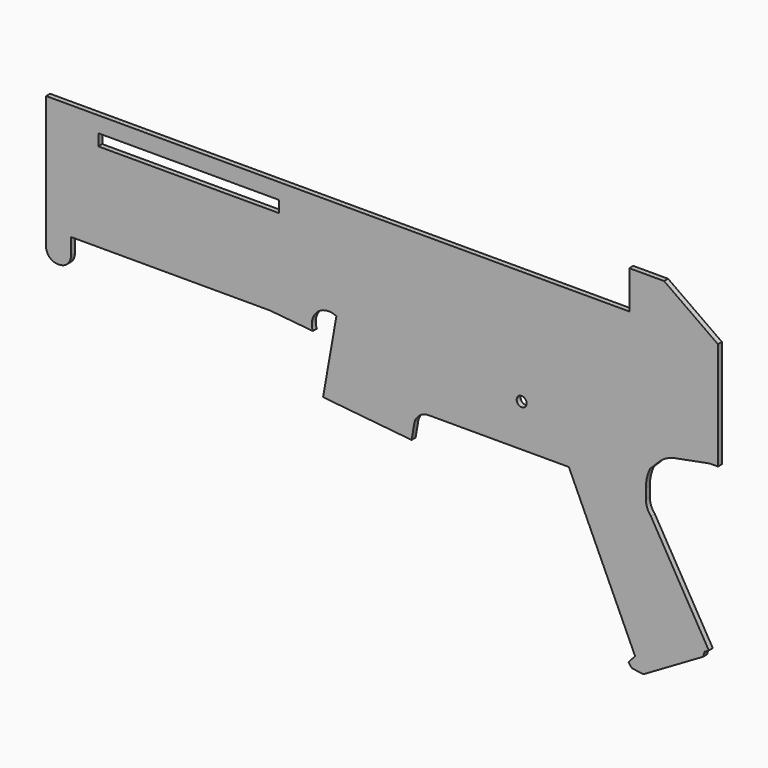
from build123d import *

# Parameters (mm, degrees)
F0_W     = 109
F0_H     = 7
F0_R     = 3
F1_DEPTH = 3


# Not quite as in the source:
# - a feature names something its author has since deleted; it is built from what else it names


with BuildPart() as f1:
    # F0 (on Front) → F1 (new body)
    with BuildSketch(Plane.XZ):
        with BuildLine():
            Line((48.4662945779, -65), (53.4662945779, -65))
            Line((53.4662945779, -65), (53.4662945779, 0))
            Line((53.4662945779, 0), (20.9662945779, 22.9999753031))
            Line((20.9662945779, 22.9999753031), (-0.0337054221, 22.9999753031))
            Line((-0.0337054221, 22.9999753031), (0, 0))
            Line((0, 0), (-352, 0))
            Line((-352, 0), (-352, -39))
            Line((-352, -39), (-352, -55.5))
            Line((-352, -55.5), (-352, -80))
            ThreePointArc((-352, -80), (-349.9497474683, -84.9497474683), (-345, -87))
            Line((-345, -87), (-344, -87))
            ThreePointArc((-344, -87), (-339.0502525317, -84.9497474683), (-337, -80))
            Line((-337, -80), (-337, -70))
            Line((-337, -70), (-217, -70))
            Line((-217, -70), (-191, -72.5))
            ThreePointArc((-191, -72.5), (-188.1802970177, -61.3925278998), (-176.8015588718, -60.0320207981))
            Line((-176.8015588718, -60.0320207981), (-179, -72.5))
            Line((-179, -72.5), (-184.8187903634, -105.5))
            Line((-184.8187903634, -105.5), (-181.3187903634, -106))
            Line((-181.3187903634, -106), (-131.43, -111.007))
            Line((-131.43, -111.007), (-129.63038537, -100.8008782668))
            ThreePointArc((-129.63038537, -100.8008782668), (-126.3267144318, -96.2419842885), (-120.9729076822, -94.5))
            Line((-120.9729076822, -94.5), (-97.5, -94.5))
            Line((-97.5, -94.5), (-36.5, -94.5))
            Line((-36.5, -94.5), (3.4662945779, -182))
            Line((3.4662945779, -182), (-0.5337054221, -186.5))
            Line((-0.5337054221, -186.5), (1.4662945779, -189))
            Line((1.4662945779, -189), (8.4662945779, -190))
            Line((8.4662945779, -190), (44.4662945779, -169))
            Line((44.4662945779, -169), (45.4662945779, -166))
            Line((45.4662945779, -166), (47.9662945779, -164.5))
            Line((47.9662945779, -164.5), (12.9662945779, -104.5))
            ThreePointArc((12.9662945779, -104.5), (10.7409562508, -100.7720018727), (9.9662945779, -96.5))
            Line((9.9662945779, -96.5), (9.9662945779, -90.5))
            ThreePointArc((9.9662945779, -90.5), (10.599163398, -84.8597429137), (12.4662945779, -79.5))
            Line((12.4662945779, -79.5), (18.4662945779, -73.5))
            ThreePointArc((18.4662945779, -73.5), (22.6544664529, -70.6263437501), (27.4662945779, -69))
            Line((27.4662945779, -69), (48.4662945779, -65))
        make_face()
        with Locations((-266, -13)):
            Rectangle(F0_W, F0_H, mode=Mode.SUBTRACT)
        with Locations((-65, -69)):
            Circle(F0_R, mode=Mode.SUBTRACT)
    extrude(amount=F1_DEPTH)


solid = f1.part
